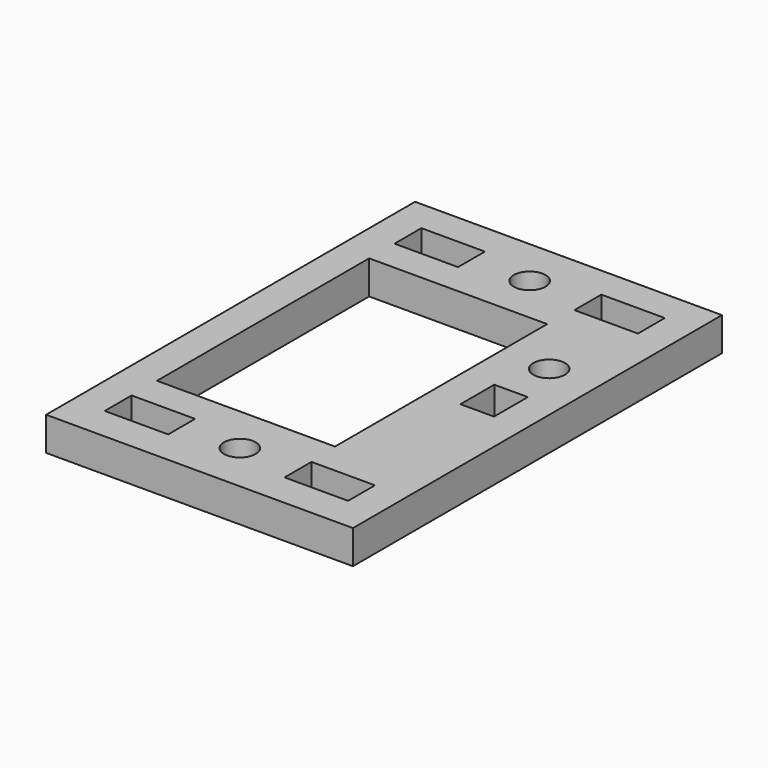
from build123d import *

# Parameters (mm, degrees)
F0_W     = 29
F0_H     = 43.5875
F0_W_2   = 6
F0_H_2   = 3.175
F0_R     = 1.5
F0_W_3   = 16.825
F0_H_3   = 25.0625
F0_W_4   = 3.175
F0_H_4   = 4
F1_DEPTH = 3.175


# Not quite as in the source:
# - a length typed as a fraction of an inch, garbled in the dataset ("3 / 203.2 mm" for 3/8 in), is restored


with BuildPart() as f1:
    # F0 (on Top) → F1 (new body)
    with BuildSketch(Plane.XY):
        with Locations((-29.1205597607, 9.4016398251)):
            Rectangle(F0_W, F0_H)
        with Locations((-37.6205597607, -7.6296101749)):
            Rectangle(F0_W_2, F0_H_2, mode=Mode.SUBTRACT)
        with Locations((-29.1205597607, -7.6296101749)):
            Circle(F0_R, mode=Mode.SUBTRACT)
        with Locations((-20.6205597607, -7.6296101749)):
            Rectangle(F0_W_2, F0_H_2, mode=Mode.SUBTRACT)
        with Locations((-32.2080597607, 9.4891398251)):
            Rectangle(F0_W_3, F0_H_3, mode=Mode.SUBTRACT)
        with Locations((-37.6205597607, 26.6078898251)):
            Rectangle(F0_W_2, F0_H_2, mode=Mode.SUBTRACT)
        with Locations((-19.2080597607, 10.0203898251)):
            Rectangle(F0_W_4, F0_H_4, mode=Mode.SUBTRACT)
        with Locations((-19.2080597607, 16.5203898251)):
            Circle(F0_R, mode=Mode.SUBTRACT)
        with Locations((-29.1205597607, 26.6078898251)):
            Circle(F0_R, mode=Mode.SUBTRACT)
        with Locations((-20.6205597607, 26.6078898251)):
            Rectangle(F0_W_2, F0_H_2, mode=Mode.SUBTRACT)
    extrude(amount=F1_DEPTH)


solid = f1.part
